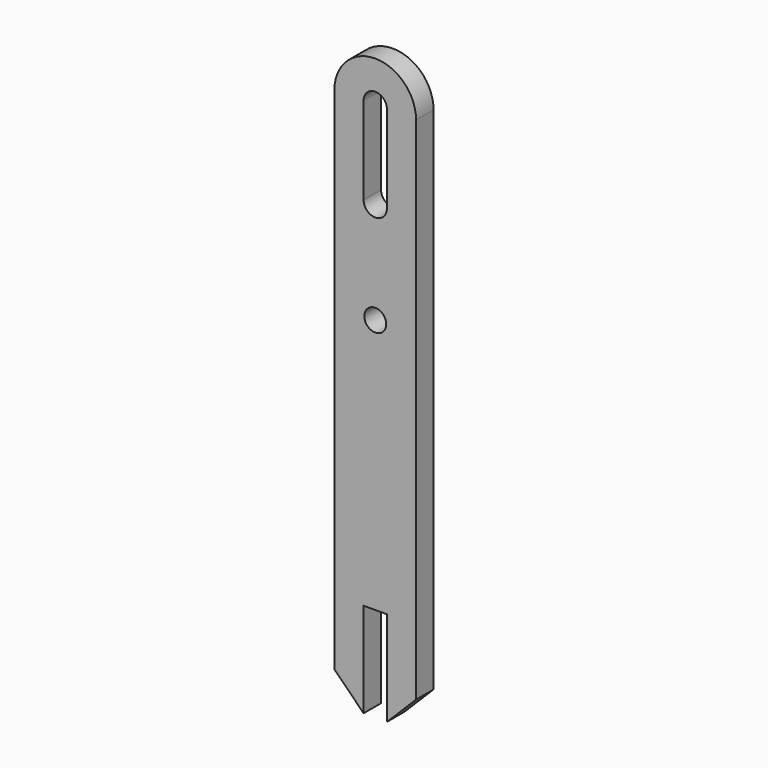
from build123d import *

# Parameters (mm, degrees)
F0_R     = 1.5
F1_DEPTH = 3
F2_SIZE  = 3.99999


# Not quite as in the source:
# - a fillet or chamfer is up to 0.001 mm smaller than in the source, because OpenCascade refuses the exact size


with BuildPart() as f1:
    # F0 (on Front) → F1 (new body)
    with BuildSketch(Plane.XZ):
        with BuildLine():
            Line((5.6, -62), (5.6, 12))
            ThreePointArc((5.6, 12), (0, 17.6), (-5.6, 12))
            Line((-5.6, 12), (-5.6, -62))
            Line((-5.6, -62), (-1.6, -62))
            Line((-1.6, -62), (-1.6, -49))
            Line((-1.6, -49), (1.6, -49))
            Line((1.6, -49), (1.6, -62))
            Line((1.6, -62), (5.6, -62))
        make_face()
        with Locations((0, -14)):
            Circle(F0_R, mode=Mode.SUBTRACT)
        with BuildLine():
            ThreePointArc((1.6, 0), (0, -1.6), (-1.6, 0))
            Line((-1.6, 0), (-1.6, 12))
            ThreePointArc((-1.6, 12), (0, 13.6), (1.6, 12))
            Line((1.6, 12), (1.6, 0))
        make_face(mode=Mode.SUBTRACT)
    extrude(amount=F1_DEPTH)

    # F2 (size 4 in the source; OpenCascade refuses exactly that, so slightly less here)
    f2_edges = [f1.edges().sort_by_distance(p)[0] for p in [
        (5.6, -1.5, -62),
        (-5.6, -1.5, -62),
    ]]
    chamfer(f2_edges, length=F2_SIZE)


solid = f1.part
